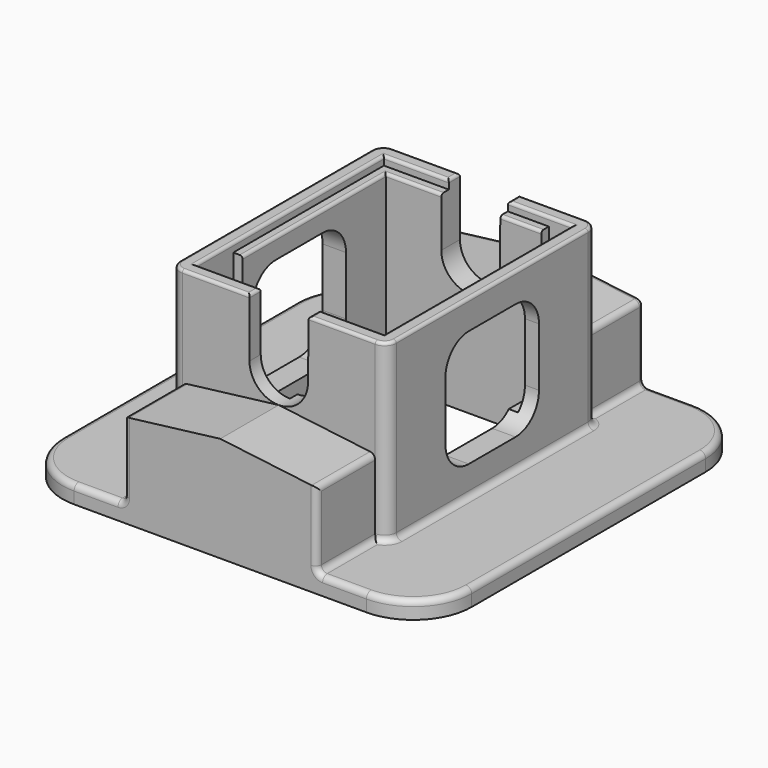
from build123d import *

# Parameters (mm, degrees)
F1_DEPTH       = 3
F3_DEPTH       = 30
F4_W           = 29
F4_H           = 37
F5_DEPTH       = 33.001
F6_W           = 32.2
F6_H           = 40.2
F7_DEPTH       = 1.5
F9_DEPTH       = 22
F10_W          = 16.1
F10_H          = 8
F11_DEPTH      = 20
F13_DEPTH      = 53.501
F13_DEPTH_BACK = 16.501
F15_DEPTH      = 57.501
F17_DEPTH      = 12.5
F19_DEPTH      = 12.5
F20_R          = 0.5
F21_R          = 1


with BuildPart() as f1:
    # F0 (on Top) → F1 (new body)
    with BuildSketch(Plane.XY):
        with BuildLine():
            Line((-25, -35), (25, -35))
            ThreePointArc((25, -35), (32.0710678119, -32.0710678119), (35, -25))
            Line((35, -25), (35, 25))
            ThreePointArc((35, 25), (32.0710678119, 32.0710678119), (25, 35))
            Line((25, 35), (-25, 35))
            ThreePointArc((-25, 35), (-32.0710678119, 32.0710678119), (-35, 25))
            Line((-35, 25), (-35, -25))
            ThreePointArc((-35, -25), (-32.0710678119, -32.0710678119), (-25, -35))
        make_face()
    extrude(amount=F1_DEPTH)

    # F2 (on face) → F3 (join)
    with BuildSketch(Plane.XY.offset(3)):
        with BuildLine():
            Line((-16.5, -22.5), (16.5, -22.5))
            ThreePointArc((16.5, -22.5), (17.9142135624, -21.9142135624), (18.5, -20.5))
            Line((18.5, -20.5), (18.5, 20.5))
            ThreePointArc((18.5, 20.5), (17.9142135624, 21.9142135624), (16.5, 22.5))
            Line((16.5, 22.5), (-16.5, 22.5))
            ThreePointArc((-16.5, 22.5), (-17.9142135624, 21.9142135624), (-18.5, 20.5))
            Line((-18.5, 20.5), (-18.5, -20.5))
            ThreePointArc((-18.5, -20.5), (-17.9142135624, -21.9142135624), (-16.5, -22.5))
        make_face()
    extrude(amount=F3_DEPTH)

    # F4 (on face) → F5 (cut, through all)
    with BuildSketch(Plane.XY.offset(33)):
        Rectangle(F4_W, F4_H)
    extrude(amount=-F5_DEPTH, mode=Mode.SUBTRACT)

    # F6 (on face) → F7 (cut)
    with BuildSketch(Plane.XY.offset(33)):
        Rectangle(F6_W, F6_H)
    extrude(amount=-F7_DEPTH, mode=Mode.SUBTRACT)

    # F8 (on face) → F9 (cut)
    with BuildSketch(Plane.XY.offset(31.5)):
        Polygon((16.1, 20.1), (12.1, 20.1), (12.1, 18.5), (14.5, 18.5), (14.5, 3.1), (16.1, 3.1), align=None)
    extrude(amount=-F9_DEPTH, mode=Mode.SUBTRACT)

    # F10 (on face) → F11 (cut)
    with BuildSketch(Plane.XY.offset(33)):
        with Locations((-8.05, -16.1)):
            Rectangle(F10_W, F10_H)
    extrude(amount=-F11_DEPTH, mode=Mode.SUBTRACT)

    # F12 (on face) → F13 (cut, two sides)
    with BuildSketch(Plane.YZ.offset(18.5)) as f13_sk:
        with BuildLine():
            Line((-5, 8.030303205), (5, 8.030303205))
            ThreePointArc((5, 8.030303205), (8.5355339059, 9.4947692991), (10, 13.030303205))
            Line((10, 13.030303205), (10, 23.030303205))
            ThreePointArc((10, 23.030303205), (8.5355339059, 26.5658371109), (5, 28.030303205))
            Line((5, 28.030303205), (-5, 28.030303205))
            ThreePointArc((-5, 28.030303205), (-8.5355339059, 26.5658371109), (-10, 23.030303205))
            Line((-10, 23.030303205), (-10, 13.030303205))
            ThreePointArc((-10, 13.030303205), (-8.5355339059, 9.4947692991), (-5, 8.030303205))
        make_face()
    extrude(amount=-F13_DEPTH, mode=Mode.SUBTRACT)
    extrude(f13_sk.sketch, amount=F13_DEPTH_BACK, mode=Mode.SUBTRACT)

    # F14 (on face) → F15 (cut, through all)
    with BuildSketch(Plane.XZ.offset(22.5)):
        with BuildLine():
            Line((-5, 33), (-5, 23))
            ThreePointArc((-5, 23), (-0.0284616664, 18.0000810073), (4.9996759734, 22.9430775894))
            Line((4.9996759734, 22.9430775894), (5.114176247, 33))
            Line((5.114176247, 33), (-5, 33))
        make_face()
    extrude(amount=-F15_DEPTH, mode=Mode.SUBTRACT)

    # F16 (on face) → F17 (join, through all)
    with BuildSketch(Plane.XZ.offset(22.5)):
        Polygon((-16.5, 15.9740547451), (-16.5, 3), (16.5, 3), (16.5, 15.9740547451), (0, 18), align=None)
    extrude(amount=F17_DEPTH)

    # F18 (on face) → F19 (join, through all)
    with BuildSketch(Plane(origin=(0, 22.5, 0), x_dir=(-1, 0, 0), z_dir=(0, 1, 0))):
        Polygon((-16.5, 15.9741357524), (-16.5, 3), (16.5, 3), (16.5, 15.9741357524), (0, 18.0000810073), align=None)
    extrude(amount=F19_DEPTH)

    # F20
    f20_edges = [f1.edges().sort_by_distance(p)[0] for p in [
        (5.114176, -21.3, 33),
        (10.607088, -20.1, 33),
        (16.1, 0, 33),
        (10.607088, 20.1, 33),
        (5.114176, 21.3, 33),
        (10.807088, 22.5, 33),
        (17.914214, 21.914214, 33),
        (18.5, 0, 33),
        (17.914214, -21.914214, 33),
        (10.807088, -22.5, 33),
        (-17.914214, -21.914214, 33),
        (-18.5, 0, 33),
        (-17.914214, 21.914214, 33),
        (-10.75, 22.5, 33),
        (-5, 21.3, 33),
        (-10.55, 20.1, 33),
        (-16.1, 0, 33),
        (-10.55, -20.1, 33),
        (-5, -21.3, 33),
        (-10.75, -22.5, 33),
        (14.5, -7.7, 31.5),
        (9.798549, -18.5, 31.5),
        (-14.5, 3.2, 31.5),
        (-9.75, 18.5, 31.5),
        (8.598549, 18.5, 31.5),
    ]]
    fillet(f20_edges, radius=F20_R)

    # F21
    f21_edges = [f1.edges().sort_by_distance(p)[0] for p in [
        (16.5, 28.75, 3),
        (8.25, 35, 16.987108),
        (-8.25, 35, 16.987108),
        (-16.5, 28.75, 3),
        (-16.5, 35, 9.487068),
        (16.5, 35, 9.487068),
        (18.5, 0, 3),
        (16.5, -28.75, 3),
        (-16.5, -28.75, 3),
        (-16.5, -35, 9.487027),
        (-16.5, 28.75, 15.974136),
        (-35, 0, 3),
        (-32.071068, 32.071068, 3),
        (-20.75, 35, 3),
        (-20.75, -35, 3),
        (-32.071068, -32.071068, 3),
        (20.75, 35, 3),
        (-16.5, -28.75, 15.974055),
        (16.5, -35, 9.487027),
        (20.75, -35, 3),
        (16.5, 28.75, 15.974136),
        (32.071068, 32.071068, 3),
        (35, 0, 3),
        (32.071068, -32.071068, 3),
        (17.914214, -21.914214, 3),
        (17.914214, 21.914214, 3),
        (16.5, -28.75, 15.974055),
    ]]
    fillet(f21_edges, radius=F21_R)


solid = f1.part
